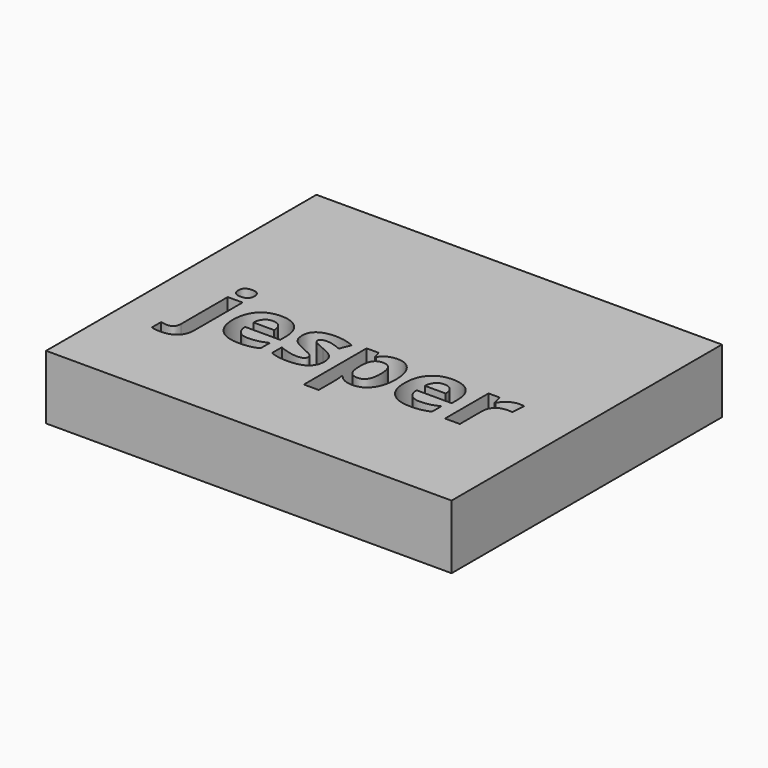
from build123d import *

# Parameters (mm, degrees)
F0_W         = 60
F0_H         = 50
F1_DEPTH     = 9.4659887254
F2_TEXT_SIZE = 14.748926171
F3_DEPTH     = 10


# Not quite as in the source:
# - Text() gives the source's letters only with a copy of the font that has no kerning and outlines rounded to 1/6400 em; it was checked with that copy


with BuildPart() as f1:
    # F0 (on Top) → F1 (new body)
    with BuildSketch(Plane.XY):
        with Locations((50.4183921177, 45.4331114888)):
            Rectangle(F0_W, F0_H)
    extrude(amount=F1_DEPTH)

    # F2 (on face) → F3 (cut)
    with BuildSketch(Plane.XY.offset(9.4659887254)):
        with Locations((27.2511336952, 35.992346704)):
            Text('jesper', F2_TEXT_SIZE, font='Open Sans', font_style=FontStyle.BOLD, text_align=(TextAlign.LEFT, TextAlign.BOTTOM))
    extrude(amount=-F3_DEPTH, mode=Mode.SUBTRACT)


solid = f1.part
